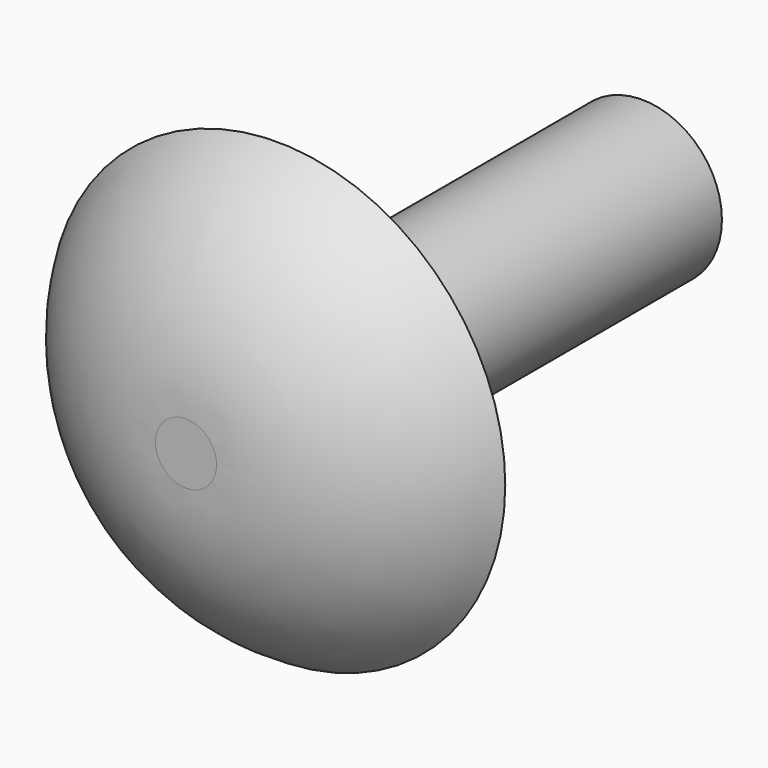
from build123d import *

# Parameters (mm, degrees)
F0_R     = 3.5
F1_DEPTH = 20
F2_R     = 10
F2_R_2   = 3.5
F3_DEPTH = 5


# Not quite as in the source:
# - a fillet or chamfer that OpenCascade refuses, or shapes differently, is made with other operations: its cross-section is extruded or revolved along the edge and cut away or added


with BuildPart() as f1:
    # F0 (on Front) → F1 (new body)
    with BuildSketch(Plane.XZ):
        Circle(F0_R)
    extrude(amount=F1_DEPTH)

    # F2 (on face) → F3 (join)
    with BuildSketch(Plane.XZ.offset(20)):
        Circle(F2_R)
        Circle(F2_R_2, mode=Mode.SUBTRACT)
        Circle(F2_R_2)
    extrude(amount=F3_DEPTH)

    # F4: fillet of radius 10 on 1 edges, made by hand

    # F4_s1 → F4_t2 (revolve, cut)
    with BuildSketch(Plane.XY):
        with BuildLine():
            ThreePointArc((10, -20), (6.3397459622, -23.6602540378), (1.3397459622, -25))
            Line((1.3397459622, -25), (10, -25))
            Line((10, -25), (10, -20))
        make_face()
    revolve(axis=Axis((0, -25, 0), (0, -1, 0)), mode=Mode.SUBTRACT)


solid = f1.part
